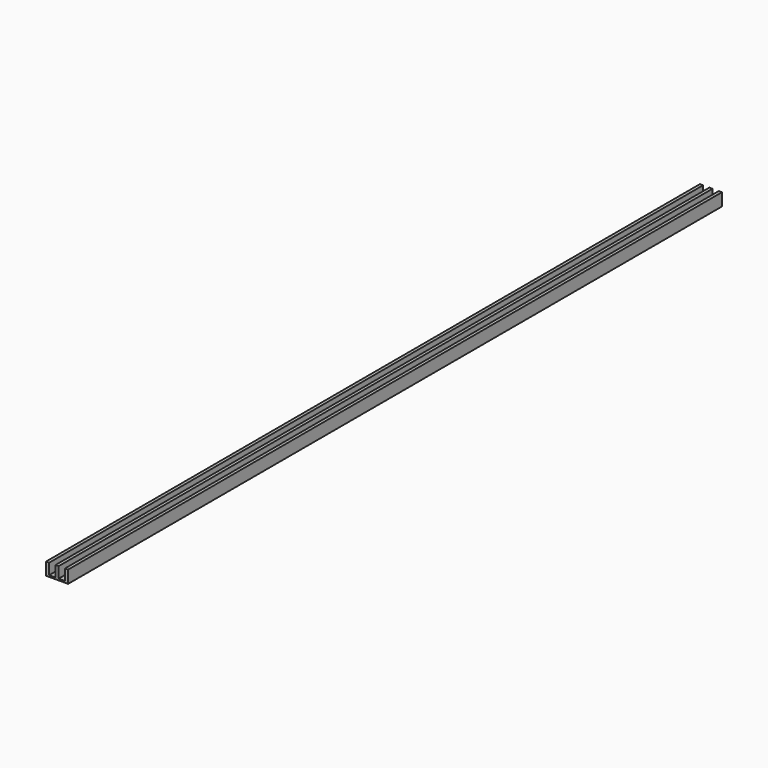
from build123d import *

# Parameters (mm, degrees)
F1_DEPTH = 1300


with BuildPart() as f1:
    # F0 (on Front) → F1 (new body, symmetric)
    with BuildSketch(Plane.XZ):
        Polygon((-25, 25), (-35, 25), (-35, -15), (35, -15), (35, 25), (25, 25), (25, -10), (5, -10), (5, 25), (-5, 25), (-5, -10), (-25, -10), align=None)
    extrude(amount=F1_DEPTH, both=True)


solid = f1.part
